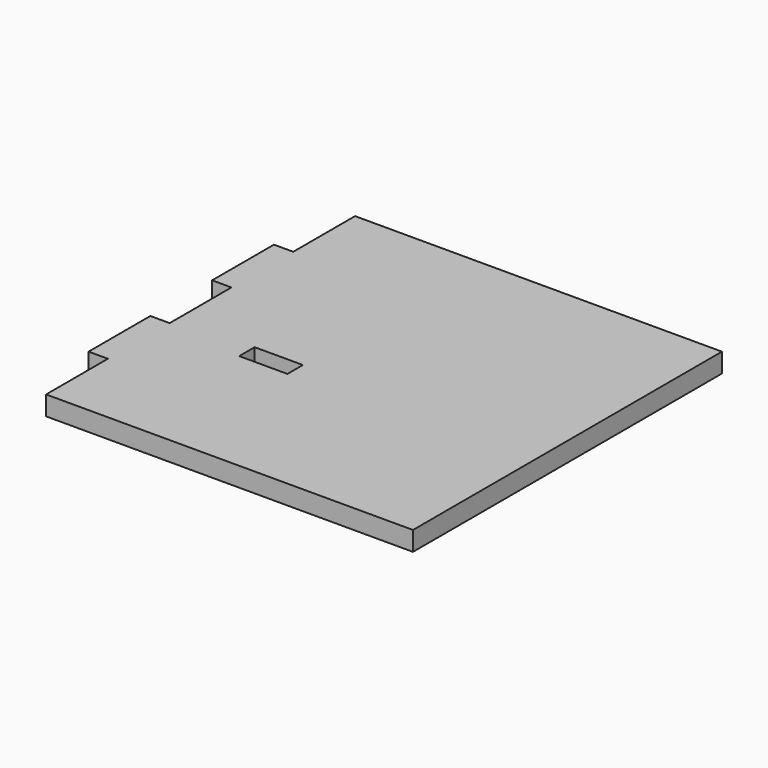
from build123d import *

# Parameters (mm, degrees)
F0_DEPTH = 2
F1_W     = 5
F1_H     = 2
F2_DEPTH = 25


# Not quite as in the source:
# - a feature names something its author has since deleted; it is built from what else it names


with BuildPart() as f0:
    # F3 (on Top) → F0 (new body)
    with BuildSketch(Plane.XY):
        Polygon((-40, 0), (-2, 0), (-2, 40), (-40, 40), (-40, 32), (-42, 32), (-42, 24), (-40, 24), (-40, 16), (-42, 16), (-42, 8), (-40, 8), align=None)
    extrude(amount=F0_DEPTH)

    # F1 (on Top) → F2 (cut)
    with BuildSketch(Plane.XY):
        with Locations((-29.5, 16)):
            Rectangle(F1_W, F1_H)
    extrude(amount=F2_DEPTH, mode=Mode.SUBTRACT)


solid = f0.part
